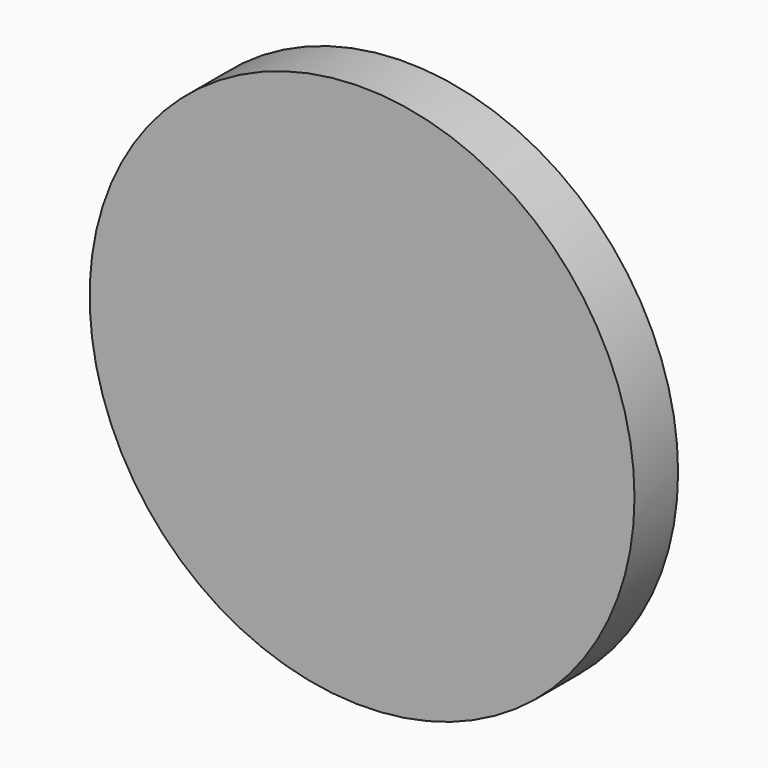
from build123d import *

# Parameters (mm, degrees)
F0_R     = 63.5
F1_DEPTH = 12.7


# Not quite as in the source:
# - the program builds the solid bodies; features that only make, move or delete a surface that nothing else refers to are left out


with BuildPart() as f1:
    # F0 (on Front) → F1 (new body)
    with BuildSketch(Plane.XZ):
        Circle(F0_R)
    extrude(amount=F1_DEPTH)


solid = f1.part
